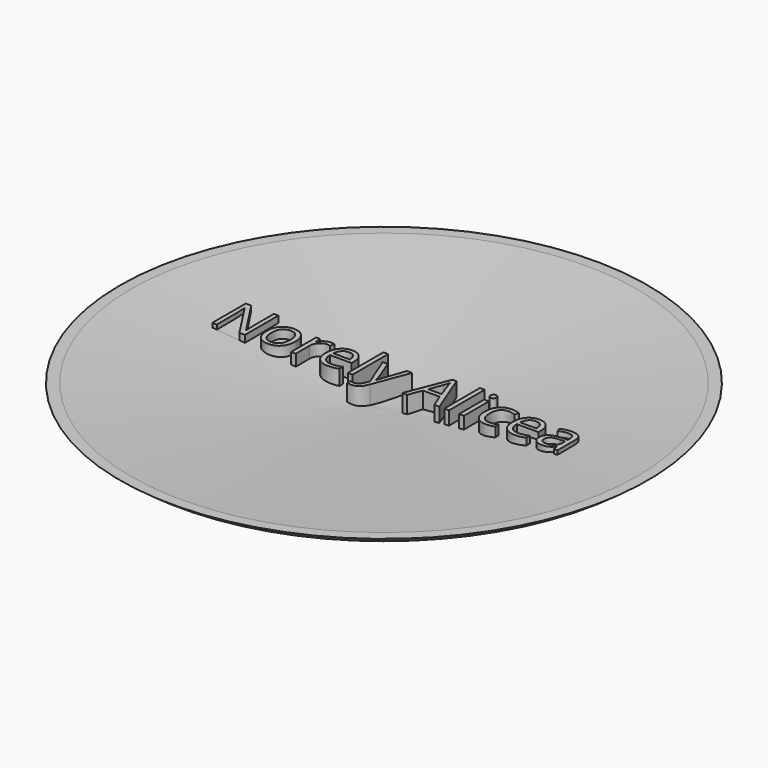
from build123d import *

# Parameters (mm, degrees)
F2_TEXT_SIZE = 15.8749999375
F3_DEPTH     = 10.414


# Not quite as in the source:
# - Text() gives the source's letters only with a copy of the font that has no kerning and outlines rounded to 1/6400 em; it was checked with that copy


with BuildPart() as f1:
    # F0 (on Front) → F1 (revolve)
    with BuildSketch(Plane.XZ):
        Polygon((-44.3691834807, 0), (0, 0), (0, 5.1954546943), (-68.6839073896, 11.2221818417), (-71.5933665633, 11.2221818417), (-68.6839073896, 9.1439997777), align=None)
    revolve(axis=Axis((0, 0, 2.5977273472), (0, 0, -1)))

    # F2 (on Top) → F3 (join)
    with BuildSketch(Plane.XY):
        with Locations((-48.1012498106, 0)):
            Text('Norely Alicea', F2_TEXT_SIZE, font='Open Sans', text_align=(TextAlign.LEFT, TextAlign.BOTTOM))
    extrude(amount=F3_DEPTH)


solid = f1.part
